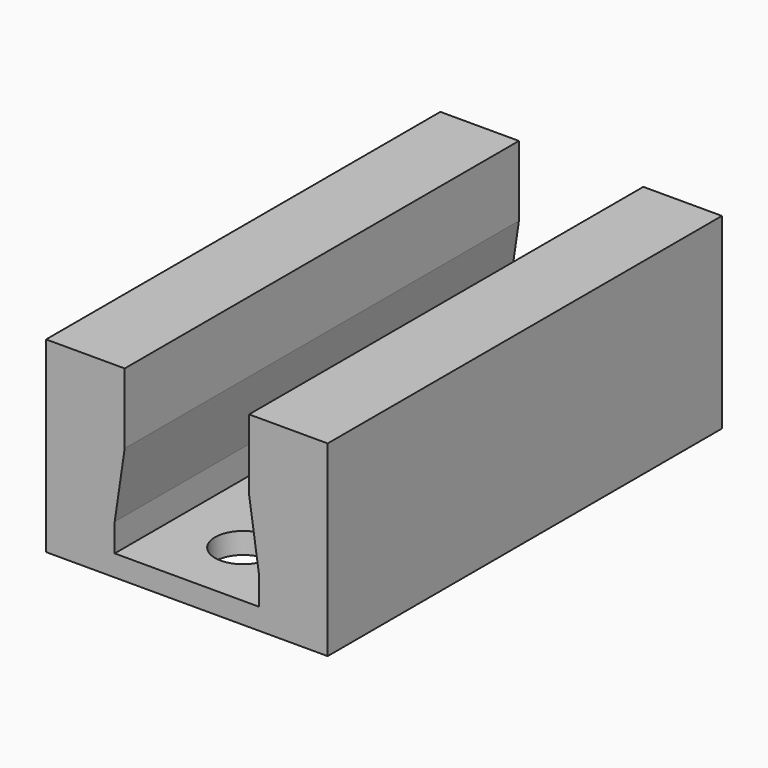
from build123d import *

# Parameters (mm, degrees)
F1_DEPTH = 35
F2_R     = 2
F3_DEPTH = 8.301
F8_DEPTH = 35.001
F9_DEPTH = 5


# Not quite as in the source:
# - a feature names something its author has since deleted; it is built from what else it names


with BuildPart() as f1:
    # F0 (on Front) → F1 (new body)
    with BuildSketch(Plane.XZ):
        Polygon((10, 4.15), (4.15, 4.15), (-4.15, 4.15), (-10, 4.15), (-10, -4.15), (-4.15, -4.15), (4.15, -4.15), (10, -4.15), align=None)
        with BuildLine():
            ThreePointArc((5.15, -1.65), (4.8571067812, -2.3571067812), (4.15, -2.65))
            Line((4.15, -2.65), (-4.15, -2.65))
            ThreePointArc((-4.15, -2.65), (-4.8571067812, -2.3571067812), (-5.15, -1.65))
            Line((-5.15, -1.65), (-5.15, 1.65))
            ThreePointArc((-5.15, 1.65), (-4.8571067812, 2.3571067812), (-4.15, 2.65))
            Line((-4.15, 2.65), (4.15, 2.65))
            ThreePointArc((4.15, 2.65), (4.8571067812, 2.3571067812), (5.15, 1.65))
            Line((5.15, 1.65), (5.15, -1.65))
        make_face(mode=Mode.SUBTRACT)
        with BuildLine():
            Line((-4.15, -2.65), (4.15, -2.65))
            ThreePointArc((4.15, -2.65), (4.8571067812, -2.3571067812), (5.15, -1.65))
            Line((5.15, -1.65), (5.15, 1.65))
            ThreePointArc((5.15, 1.65), (4.8571067812, 2.3571067812), (4.15, 2.65))
            Line((4.15, 2.65), (-4.15, 2.65))
            ThreePointArc((-4.15, 2.65), (-4.8571067812, 2.3571067812), (-5.15, 1.65))
            Line((-5.15, 1.65), (-5.15, -1.65))
            ThreePointArc((-5.15, -1.65), (-4.8571067812, -2.3571067812), (-4.15, -2.65))
        make_face()
    extrude(amount=F1_DEPTH)

    # F2 (on face) → F3 (cut, through all)
    with BuildSketch(Plane.XY.offset(4.15)):
        with Locations((0, -5)):
            Circle(F2_R)
        with Locations((0, -30)):
            Circle(F2_R)
    extrude(amount=-F3_DEPTH, mode=Mode.SUBTRACT)

    # F7 (on offset) → F8 (cut, through all)
    with BuildSketch(Plane.XZ.offset(35)):
        Polygon((-5.1262229681, -2.646596171), (0, -2.646596171), (5.1262229681, -2.646596171), (5.1262229681, -0.6600963534), (4.3867812492, 4.353403829), (0, 4.353403829), (-4.3867812492, 4.353403829), (-5.1262229681, -0.6600963534), align=None)
    extrude(amount=-F8_DEPTH, mode=Mode.SUBTRACT)

    # F9 (add): faces of the model
    f9_faces = [f1.faces().sort_by_distance(p)[0] for p in [
        (-7.2083906517, -17.5, 4.15),
        (7.2083906517, -17.5, 4.15),
    ]]
    extrude(f9_faces, amount=F9_DEPTH)


solid = f1.part
